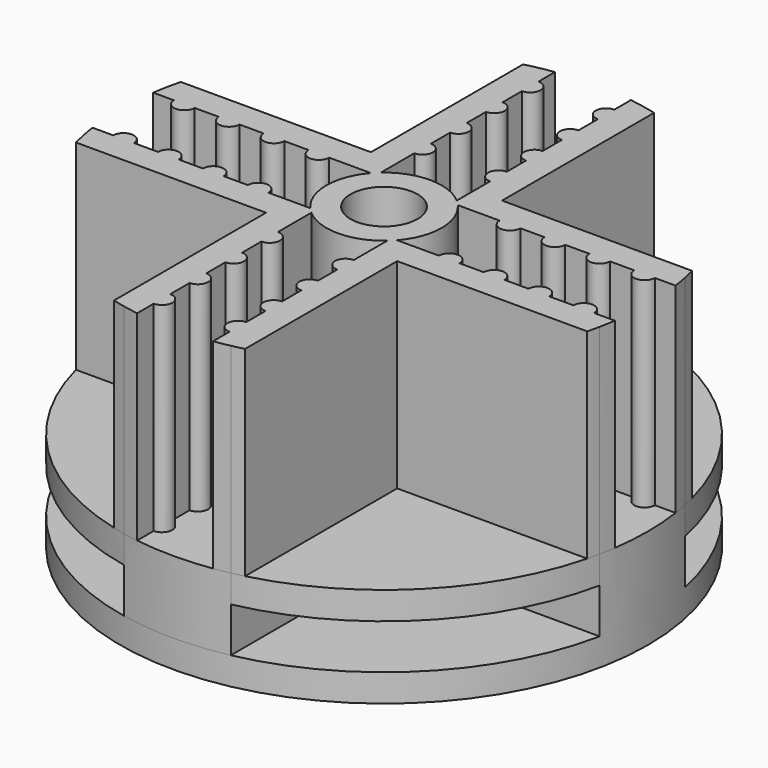
from build123d import *
from build123d import SkipClean  # not in build123d's __all__

# Parameters (mm, degrees)
F0_R      = 19.431
F1_DEPTH  = 2.032
F3_DEPTH  = 5.334
F5_DEPTH  = 14.732
F6_R      = 4.2469525028
F6_R_2    = 2.4689525028
F7_DEPTH  = 14.732
F9_DEPTH  = 2.032
F11_DEPTH = 14.732


# Not quite as in the source:
# - after a boolean that leaves OpenCascade's solid faulty, fix() repairs it


with BuildPart() as f1:
    # F0 (on Top) → F1 (new body)
    with BuildSketch(Plane.XY):
        Circle(F0_R)
    extrude(amount=F1_DEPTH)

    # F2 (on face) → F3 (join)
    with BuildSketch(Plane.XY.offset(2.032)):
        with BuildLine():
            Line((3.937, 3.937), (3.937, 19.0279739331))
            ThreePointArc((3.937, 19.0279739331), (0, 19.431), (-3.937, 19.0279739331))
            Line((-3.937, 19.0279739331), (-3.937, 3.937))
            Line((-3.937, 3.937), (-19.0279739331, 3.937))
            ThreePointArc((-19.0279739331, 3.937), (-19.431, 0), (-19.0279739331, -3.937))
            Line((-19.0279739331, -3.937), (-3.937, -3.937))
            Line((-3.937, -3.937), (-3.937, -19.0279739331))
            ThreePointArc((-3.937, -19.0279739331), (0, -19.431), (3.937, -19.0279739331))
            Line((3.937, -19.0279739331), (3.937, -3.937))
            Line((3.937, -3.937), (19.0279739331, -3.937))
            ThreePointArc((19.0279739331, -3.937), (19.431, 0), (19.0279739331, 3.937))
            Line((19.0279739331, 3.937), (3.937, 3.937))
        make_face()
    extrude(amount=F3_DEPTH)

    # F4 (on face) → F5 (join)
    with BuildSketch(Plane.XY.offset(7.366)):
        with BuildLine():
            ThreePointArc((3.937, 19.0279739331), (3.3670017313, 19.1370598667), (2.794, 19.2290749908))
            Line((2.794, 19.2290749908), (2.794, 2.794))
            Line((2.794, 2.794), (19.2290749908, 2.794))
            ThreePointArc((19.2290749908, 2.794), (19.1370598667, 3.3670017313), (19.0279739331, 3.937))
            ThreePointArc((19.0279739331, 3.937), (18.9302833655, 4.3827083751), (18.822154101, 4.826))
            Line((18.822154101, 4.826), (4.826, 4.826))
            Line((4.826, 4.826), (4.826, 18.822154101))
            ThreePointArc((4.826, 18.822154101), (4.3827083751, 18.9302833655), (3.937, 19.0279739331))
        make_face()
        with BuildLine():
            ThreePointArc((-3.937, 19.0279739331), (-4.3827083751, 18.9302833655), (-4.826, 18.822154101))
            Line((-4.826, 18.822154101), (-4.826, 4.826))
            Line((-4.826, 4.826), (-18.822154101, 4.826))
            ThreePointArc((-18.822154101, 4.826), (-18.9302833655, 4.3827083751), (-19.0279739331, 3.937))
            ThreePointArc((-19.0279739331, 3.937), (-19.1370598667, 3.3670017313), (-19.2290749908, 2.794))
            Line((-19.2290749908, 2.794), (-2.794, 2.794))
            Line((-2.794, 2.794), (-2.794, 19.2290749908))
            ThreePointArc((-2.794, 19.2290749908), (-3.3670017313, 19.1370598667), (-3.937, 19.0279739331))
        make_face()
        with BuildLine():
            ThreePointArc((-19.0279739331, -3.937), (-18.9302833655, -4.3827083751), (-18.822154101, -4.826))
            Line((-18.822154101, -4.826), (-4.826, -4.826))
            Line((-4.826, -4.826), (-4.826, -18.822154101))
            ThreePointArc((-4.826, -18.822154101), (-4.3827083751, -18.9302833655), (-3.937, -19.0279739331))
            ThreePointArc((-3.937, -19.0279739331), (-3.3670017313, -19.1370598667), (-2.794, -19.2290749908))
            Line((-2.794, -19.2290749908), (-2.794, -2.794))
            Line((-2.794, -2.794), (-19.2290749908, -2.794))
            ThreePointArc((-19.2290749908, -2.794), (-19.1370598667, -3.3670017313), (-19.0279739331, -3.937))
        make_face()
        with BuildLine():
            ThreePointArc((3.937, -19.0279739331), (4.3827083751, -18.9302833655), (4.826, -18.822154101))
            Line((4.826, -18.822154101), (4.826, -4.826))
            Line((4.826, -4.826), (18.822154101, -4.826))
            ThreePointArc((18.822154101, -4.826), (18.9302833655, -4.3827083751), (19.0279739331, -3.937))
            ThreePointArc((19.0279739331, -3.937), (19.1370598667, -3.3670017313), (19.2290749908, -2.794))
            Line((19.2290749908, -2.794), (2.794, -2.794))
            Line((2.794, -2.794), (2.794, -19.2290749908))
            ThreePointArc((2.794, -19.2290749908), (3.3670017313, -19.1370598667), (3.937, -19.0279739331))
        make_face()
    extrude(amount=F5_DEPTH)

    # F6 (on face) → F7 (join, through all)
    with BuildSketch(Plane.XY.offset(7.366)):
        Circle(F6_R)
        Circle(F6_R_2, mode=Mode.SUBTRACT)
    extrude(amount=F7_DEPTH)

    # F8 (on face) → F9 (join)
    with BuildSketch(Plane(origin=(0, 0, 7.366), x_dir=(1, 0, 0), z_dir=(0, 0, -1))):
        with BuildLine():
            Line((-3.937, 3.937), (-3.937, 19.0279739331))
            ThreePointArc((-3.937, 19.0279739331), (-13.7397918652, 13.7397918652), (-19.0279739331, 3.937))
            Line((-19.0279739331, 3.937), (-3.937, 3.937))
        make_face()
        with BuildLine():
            ThreePointArc((-19.0279739331, -3.937), (-13.7397918652, -13.7397918652), (-3.937, -19.0279739331))
            Line((-3.937, -19.0279739331), (-3.937, -3.937))
            Line((-3.937, -3.937), (-19.0279739331, -3.937))
        make_face()
        with BuildLine():
            ThreePointArc((3.937, -19.0279739331), (13.7397918652, -13.7397918652), (19.0279739331, -3.937))
            Line((19.0279739331, -3.937), (3.937, -3.937))
            Line((3.937, -3.937), (3.937, -19.0279739331))
        make_face()
        with BuildLine():
            ThreePointArc((19.0279739331, 3.937), (13.7397918652, 13.7397918652), (3.937, 19.0279739331))
            Line((3.937, 19.0279739331), (3.937, 3.937))
            Line((3.937, 3.937), (19.0279739331, 3.937))
        make_face()
    with SkipClean():  # cleaning this boolean's faces spoils the solid; the shape is the same uncleaned
        extrude(amount=F9_DEPTH)

    # F10 (on face) → F11 (join, through all)
    with BuildSketch(Plane.XY.offset(22.098)):
        with BuildLine():
            Line((16.1810749908, -2.794), (17.7050749908, -2.794))
            ThreePointArc((17.7050749908, -2.794), (16.9430749908, -2.032), (16.1810749908, -2.794))
        make_face()
        with BuildLine():
            Line((12.8790749908, -2.794), (14.4030749908, -2.794))
            ThreePointArc((14.4030749908, -2.794), (13.6410749908, -2.032), (12.8790749908, -2.794))
        make_face()
        with BuildLine():
            Line((9.5770749908, -2.794), (11.1010749908, -2.794))
            ThreePointArc((11.1010749908, -2.794), (10.3390749908, -2.032), (9.5770749908, -2.794))
        make_face()
        with BuildLine():
            Line((6.2750749908, -2.794), (7.7990749908, -2.794))
            ThreePointArc((7.7990749908, -2.794), (7.0370749908, -2.032), (6.2750749908, -2.794))
        make_face()
        with BuildLine():
            ThreePointArc((16.1810749908, 2.794), (16.9430749908, 2.032), (17.7050749908, 2.794))
            Line((17.7050749908, 2.794), (16.1810749908, 2.794))
        make_face()
        with BuildLine():
            ThreePointArc((6.2750749908, 2.794), (7.0370749908, 2.032), (7.7990749908, 2.794))
            Line((7.7990749908, 2.794), (6.2750749908, 2.794))
        make_face()
        with BuildLine():
            ThreePointArc((12.8790749908, 2.794), (13.6410749908, 2.032), (14.4030749908, 2.794))
            Line((14.4030749908, 2.794), (12.8790749908, 2.794))
        make_face()
        with BuildLine():
            ThreePointArc((9.5770749908, 2.794), (10.3390749908, 2.032), (11.1010749908, 2.794))
            Line((11.1010749908, 2.794), (9.5770749908, 2.794))
        make_face()
        with BuildLine():
            Line((2.794, 9.5770749908), (2.794, 11.1010749908))
            ThreePointArc((2.794, 11.1010749908), (2.032, 10.3390749908), (2.794, 9.5770749908))
        make_face()
        with BuildLine():
            ThreePointArc((-2.794, 9.5770749908), (-2.032, 10.3390749908), (-2.794, 11.1010749908))
            Line((-2.794, 11.1010749908), (-2.794, 9.5770749908))
        make_face()
        with BuildLine():
            Line((2.794, 6.2750749908), (2.794, 7.7990749908))
            ThreePointArc((2.794, 7.7990749908), (2.032, 7.0370749908), (2.794, 6.2750749908))
        make_face()
        with BuildLine():
            Line((2.794, 16.1810749908), (2.794, 17.7050749908))
            ThreePointArc((2.794, 17.7050749908), (2.032, 16.9430749908), (2.794, 16.1810749908))
        make_face()
        with BuildLine():
            ThreePointArc((-2.794, 16.1810749908), (-2.032, 16.9430749908), (-2.794, 17.7050749908))
            Line((-2.794, 17.7050749908), (-2.794, 16.1810749908))
        make_face()
        with BuildLine():
            ThreePointArc((-2.794, 6.2750749908), (-2.032, 7.0370749908), (-2.794, 7.7990749908))
            Line((-2.794, 7.7990749908), (-2.794, 6.2750749908))
        make_face()
        with BuildLine():
            Line((2.794, 12.8790749908), (2.794, 14.4030749908))
            ThreePointArc((2.794, 14.4030749908), (2.032, 13.6410749908), (2.794, 12.8790749908))
        make_face()
        with BuildLine():
            ThreePointArc((-2.794, 12.8790749908), (-2.032, 13.6410749908), (-2.794, 14.4030749908))
            Line((-2.794, 14.4030749908), (-2.794, 12.8790749908))
        make_face()
        with BuildLine():
            Line((-9.5770749908, 2.794), (-11.1010749908, 2.794))
            ThreePointArc((-11.1010749908, 2.794), (-10.3390749908, 2.032), (-9.5770749908, 2.794))
        make_face()
        with BuildLine():
            ThreePointArc((-9.5770749908, -2.794), (-10.3390749908, -2.032), (-11.1010749908, -2.794))
            Line((-11.1010749908, -2.794), (-9.5770749908, -2.794))
        make_face()
        with BuildLine():
            Line((-6.2750749908, 2.794), (-7.7990749908, 2.794))
            ThreePointArc((-7.7990749908, 2.794), (-7.0370749908, 2.032), (-6.2750749908, 2.794))
        make_face()
        with BuildLine():
            Line((-16.1810749908, 2.794), (-17.7050749908, 2.794))
            ThreePointArc((-17.7050749908, 2.794), (-16.9430749908, 2.032), (-16.1810749908, 2.794))
        make_face()
        with BuildLine():
            ThreePointArc((-16.1810749908, -2.794), (-16.9430749908, -2.032), (-17.7050749908, -2.794))
            Line((-17.7050749908, -2.794), (-16.1810749908, -2.794))
        make_face()
        with BuildLine():
            ThreePointArc((-6.2750749908, -2.794), (-7.0370749908, -2.032), (-7.7990749908, -2.794))
            Line((-7.7990749908, -2.794), (-6.2750749908, -2.794))
        make_face()
        with BuildLine():
            Line((-12.8790749908, 2.794), (-14.4030749908, 2.794))
            ThreePointArc((-14.4030749908, 2.794), (-13.6410749908, 2.032), (-12.8790749908, 2.794))
        make_face()
        with BuildLine():
            ThreePointArc((-12.8790749908, -2.794), (-13.6410749908, -2.032), (-14.4030749908, -2.794))
            Line((-14.4030749908, -2.794), (-12.8790749908, -2.794))
        make_face()
        with BuildLine():
            Line((-2.794, -9.5770749908), (-2.794, -11.1010749908))
            ThreePointArc((-2.794, -11.1010749908), (-2.032, -10.3390749908), (-2.794, -9.5770749908))
        make_face()
        with BuildLine():
            ThreePointArc((2.794, -9.5770749908), (2.032, -10.3390749908), (2.794, -11.1010749908))
            Line((2.794, -11.1010749908), (2.794, -9.5770749908))
        make_face()
        with BuildLine():
            Line((-2.794, -6.2750749908), (-2.794, -7.7990749908))
            ThreePointArc((-2.794, -7.7990749908), (-2.032, -7.0370749908), (-2.794, -6.2750749908))
        make_face()
        with BuildLine():
            Line((-2.794, -16.1810749908), (-2.794, -17.7050749908))
            ThreePointArc((-2.794, -17.7050749908), (-2.032, -16.9430749908), (-2.794, -16.1810749908))
        make_face()
        with BuildLine():
            ThreePointArc((2.794, -16.1810749908), (2.032, -16.9430749908), (2.794, -17.7050749908))
            Line((2.794, -17.7050749908), (2.794, -16.1810749908))
        make_face()
        with BuildLine():
            ThreePointArc((2.794, -6.2750749908), (2.032, -7.0370749908), (2.794, -7.7990749908))
            Line((2.794, -7.7990749908), (2.794, -6.2750749908))
        make_face()
        with BuildLine():
            Line((-2.794, -12.8790749908), (-2.794, -14.4030749908))
            ThreePointArc((-2.794, -14.4030749908), (-2.032, -13.6410749908), (-2.794, -12.8790749908))
        make_face()
        with BuildLine():
            ThreePointArc((2.794, -12.8790749908), (2.032, -13.6410749908), (2.794, -14.4030749908))
            Line((2.794, -14.4030749908), (2.794, -12.8790749908))
        make_face()
    extrude(amount=-F11_DEPTH)

    add(f1.part.fix(), mode=Mode.REPLACE)


solid = f1.part
